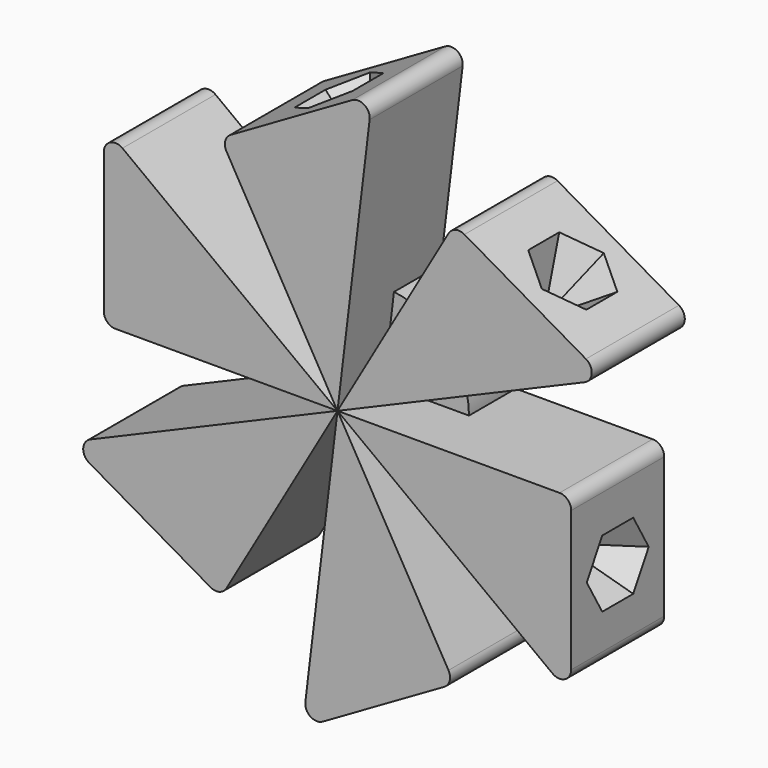
from build123d import *

# Parameters (mm, degrees)
F1_DEPTH = 50.546
F2_R     = 5.08
F5_COUNT = 6
F6_R     = 37.0441580262
F7_DEPTH = 25.4


# Not quite as in the source:
# - an extrude whose draft closes it to a point is written as a loft to that point


with BuildPart() as f1:
    # F0 (on Front) → F1 (new body)
    with BuildSketch(Plane.XZ):
        Polygon((56.3211010993, 27.6779612722), (-45.2788989007, 27.6779612722), (56.3211010993, -48.5220387278), align=None)
    extrude(amount=F1_DEPTH)

    # F2
    f2_edges = [f1.edges().sort_by_distance(p)[0] for p in [
        (56.321101, -25.273, -48.522039),
        (56.321101, -25.273, 27.677961),
    ]]
    fillet(f2_edges, radius=F2_R)

    # F3 (on face) → F4 section 0
    with BuildSketch(Plane.YZ.offset(56.3211010993), mode=Mode.PRIVATE) as f4_s0:
        Polygon((-16.8529431718, 6.1591384001), (-33.6930568282, 6.1591384001), (-42.1131136565, -8.424827829), (-33.6930568282, -23.0087940581), (-16.8529431718, -23.0087940581), (-8.4328863435, -8.424827829), align=None)
    loft([f4_s0.sketch, Vertex(31.0609306146, -25.273, -8.424827829)], ruled=True, mode=Mode.SUBTRACT)


with BuildPart() as f5_1:
    # F5: instance of F1
    add(f1.part.rotate(Axis((-45.2788989007, -25.273, 27.6779612722), (0, 1, 0)), 1 * 360 / F5_COUNT))


with BuildPart() as f5_2:
    # F5: instance of F1
    add(f1.part.rotate(Axis((-45.2788989007, -25.273, 27.6779612722), (0, 1, 0)), 2 * 360 / F5_COUNT))


with BuildPart() as f5_3:
    # F5: instance of F1
    add(f1.part.rotate(Axis((-45.2788989007, -25.273, 27.6779612722), (0, 1, 0)), 3 * 360 / F5_COUNT))


with BuildPart() as f5_4:
    # F5: instance of F1
    add(f1.part.rotate(Axis((-45.2788989007, -25.273, 27.6779612722), (0, 1, 0)), 4 * 360 / F5_COUNT))


with BuildPart() as f5_5:
    # F5: instance of F1
    add(f1.part.rotate(Axis((-45.2788989007, -25.273, 27.6779612722), (0, 1, 0)), 5 * 360 / F5_COUNT))


with BuildPart() as f7:
    # F6 (on Front) → F7 (new body)
    with BuildSketch(Plane.XZ):
        with Locations((-45.2788989007, 27.6779612722)):
            Circle(F6_R)
    extrude(amount=F7_DEPTH)


solid = Compound([f1.part, f5_1.part, f5_2.part, f5_3.part, f5_4.part, f5_5.part, f7.part])
